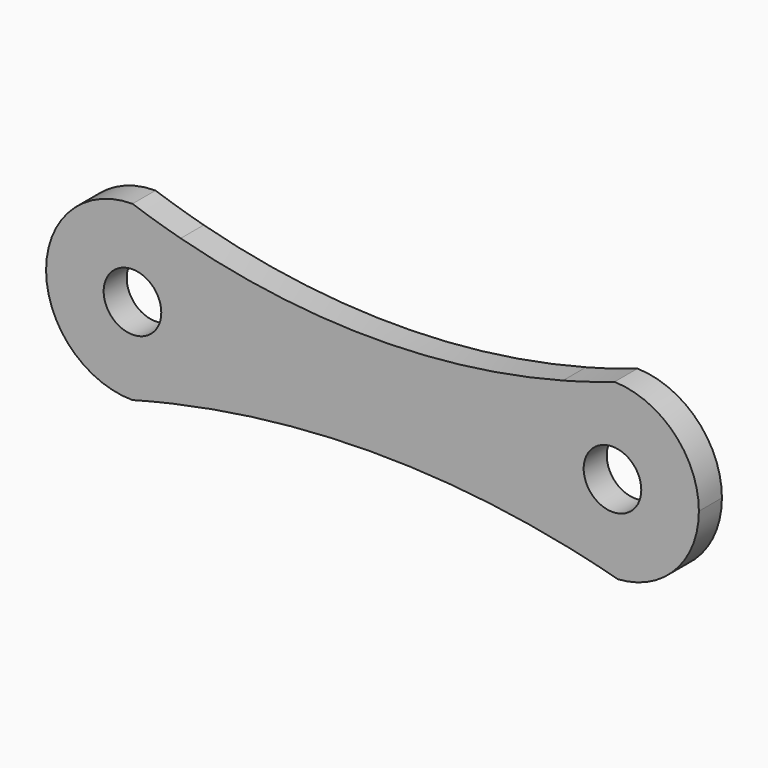
from build123d import *

# Parameters (mm, degrees)
F0_R     = 3
F1_DEPTH = 3


with BuildPart() as f1:
    # F0 (on Front) → F1 (new body)
    with BuildSketch(Plane.XZ):
        with BuildLine():
            ThreePointArc((5.0238306032, 7.4673372811), (2.4989245726, 8.1910870463), (0, 9))
            ThreePointArc((0, 9), (-9, 0), (0, -9))
            ThreePointArc((0, -9), (2.0891997796, -8.459259966), (4.1899294664, -7.9652050235))
            ThreePointArc((4.1899294664, -7.9652050235), (7.7041990238, -4.6524528371), (9, 0))
            ThreePointArc((9, 0), (7.944006402, 4.2299837217), (5.0238306032, 7.4673372811))
        make_face()
        Circle(F0_R, mode=Mode.SUBTRACT)
        with BuildLine():
            ThreePointArc((44.8388245261, 7.3730772224), (24.9251697087, 4.8191586202), (5.0238306032, 7.4673372811))
            ThreePointArc((5.0238306032, 7.4673372811), (7.944006402, 4.2299837217), (9, 0))
            ThreePointArc((9, 0), (7.7041990238, -4.6524528371), (4.1899294664, -7.9652050235))
            ThreePointArc((4.1899294664, -7.9652050235), (24.7899854963, -5.6356561903), (45.4138690609, -7.7438622799))
            ThreePointArc((45.4138690609, -7.7438622799), (41.0065045418, -0.3421102804), (44.8388245261, 7.3730772224))
        make_face()
        with BuildLine():
            ThreePointArc((50.2100552652, 8.9975483764), (47.5391507079, 8.1366722514), (44.8388245261, 7.3730772224))
            ThreePointArc((44.8388245261, 7.3730772224), (41.0065045418, -0.3421102804), (45.4138690609, -7.7438622799))
            ThreePointArc((45.4138690609, -7.7438622799), (47.9935464321, -8.3282112662), (50.5563037426, -8.9827905545))
            ThreePointArc((50.5563037426, -8.9827905545), (56.5576952386, -6.16414091), (59, 0))
            ThreePointArc((59, 0), (56.4377984353, 6.2892568167), (50.2100552652, 8.9975483764))
        make_face()
        with Locations((50, 0)):
            Circle(F0_R, mode=Mode.SUBTRACT)
    extrude(amount=F1_DEPTH)


solid = f1.part
